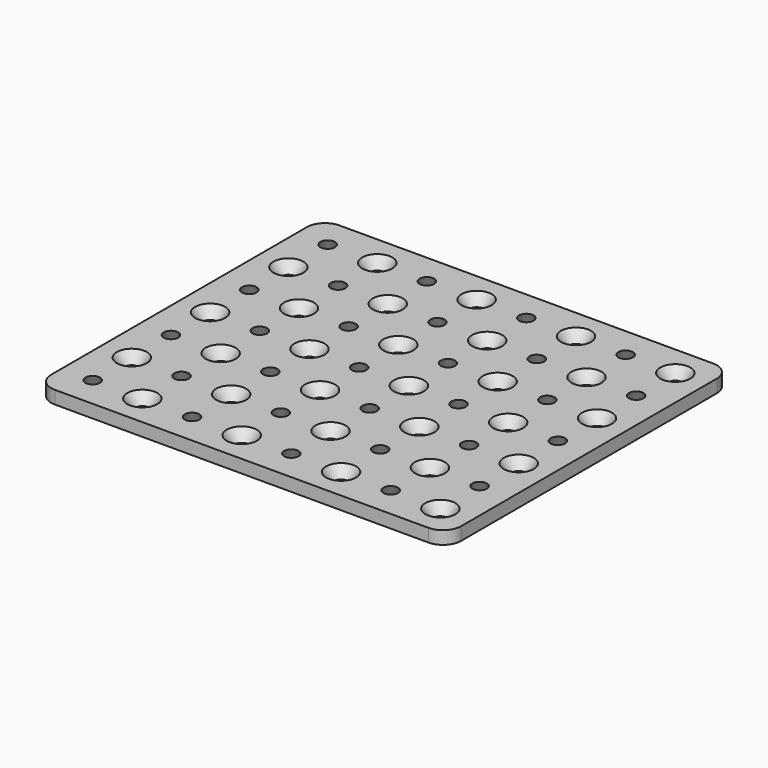
from build123d import *

# Parameters (mm, degrees)
F0_W        = 79
F0_H        = 68.58
F0_R        = 1.397
F1_DEPTH    = 1.25
F2_R        = 3.5
F3_SIZE2    = 2.49999
F3_SIZE     = 1.49999
F4_SIZE2    = 1.5
F4_SIZE     = 2
F4_2_SIZE2  = 1.5
F4_2_SIZE   = 2
F4_3_SIZE2  = 1.5
F4_3_SIZE   = 2
F4_4_SIZE2  = 1.5
F4_4_SIZE   = 2
F4_5_SIZE2  = 1.5
F4_5_SIZE   = 2
F4_6_SIZE2  = 1.5
F4_6_SIZE   = 2
F4_7_SIZE2  = 1.5
F4_7_SIZE   = 2
F4_8_SIZE2  = 1.5
F4_8_SIZE   = 2
F4_9_SIZE2  = 1.5
F4_9_SIZE   = 2
F4_10_SIZE2 = 1.5
F4_10_SIZE  = 2
F4_11_SIZE2 = 1.5
F4_11_SIZE  = 2
F4_12_SIZE2 = 1.5
F4_12_SIZE  = 2
F4_13_SIZE2 = 1.5
F4_13_SIZE  = 2
F4_14_SIZE2 = 1.5
F4_14_SIZE  = 2
F4_15_SIZE2 = 1.5
F4_15_SIZE  = 2
F4_16_SIZE2 = 1.5
F4_16_SIZE  = 2
F4_17_SIZE2 = 1.5
F4_17_SIZE  = 2
F4_18_SIZE2 = 1.5
F4_18_SIZE  = 2
F4_19_SIZE2 = 1.5
F4_19_SIZE  = 2
F4_20_SIZE2 = 1.5
F4_20_SIZE  = 2
F4_21_SIZE2 = 1.5
F4_21_SIZE  = 2
F4_22_SIZE2 = 1.5
F4_22_SIZE  = 2
F4_23_SIZE2 = 1.5
F4_23_SIZE  = 2
F4_24_SIZE2 = 1.5
F4_24_SIZE  = 2
F4_25_SIZE2 = 1.5
F4_25_SIZE  = 2
F4_26_SIZE2 = 1.5
F4_26_SIZE  = 2
F4_27_SIZE2 = 1.5
F4_27_SIZE  = 2
F4_28_SIZE2 = 1.5
F4_28_SIZE  = 2


# Not quite as in the source:
# - a fillet or chamfer is up to 0.001 mm smaller than in the source, because OpenCascade refuses the exact size


with BuildPart() as f1:
    # F0 (on Top) → F1 (new body, symmetric)
    with BuildSketch(Plane.XY):
        Rectangle(F0_W, F0_H)
        with Locations((-33.5, -28.29)):
            Circle(F0_R, mode=Mode.SUBTRACT)
        with Locations((-23.9285714286, -28.29)):
            Circle(F0_R, mode=Mode.SUBTRACT)
        with Locations((-33.5, -18.86)):
            Circle(F0_R, mode=Mode.SUBTRACT)
        with Locations((-23.9285714286, -18.86)):
            Circle(F0_R, mode=Mode.SUBTRACT)
        with Locations((-14.3571428571, -28.29)):
            Circle(F0_R, mode=Mode.SUBTRACT)
        with Locations((-4.7857142857, -28.29)):
            Circle(F0_R, mode=Mode.SUBTRACT)
        with Locations((-14.3571428571, -18.86)):
            Circle(F0_R, mode=Mode.SUBTRACT)
        with Locations((-4.7857142857, -18.86)):
            Circle(F0_R, mode=Mode.SUBTRACT)
        with Locations((-33.5, -9.43)):
            Circle(F0_R, mode=Mode.SUBTRACT)
        with Locations((-23.9285714286, -9.43)):
            Circle(F0_R, mode=Mode.SUBTRACT)
        with Locations((-14.3571428571, -9.43)):
            Circle(F0_R, mode=Mode.SUBTRACT)
        with Locations((-4.7857142857, -9.43)):
            Circle(F0_R, mode=Mode.SUBTRACT)
        with Locations((4.7857142857, -28.29)):
            Circle(F0_R, mode=Mode.SUBTRACT)
        with Locations((14.3571428571, -28.29)):
            Circle(F0_R, mode=Mode.SUBTRACT)
        with Locations((4.7857142857, -18.86)):
            Circle(F0_R, mode=Mode.SUBTRACT)
        with Locations((14.3571428571, -18.86)):
            Circle(F0_R, mode=Mode.SUBTRACT)
        with Locations((23.9285714286, -28.29)):
            Circle(F0_R, mode=Mode.SUBTRACT)
        with Locations((33.5, -28.29)):
            Circle(F0_R, mode=Mode.SUBTRACT)
        with Locations((23.9285714286, -18.86)):
            Circle(F0_R, mode=Mode.SUBTRACT)
        with Locations((33.5, -18.86)):
            Circle(F0_R, mode=Mode.SUBTRACT)
        with Locations((4.7857142857, -9.43)):
            Circle(F0_R, mode=Mode.SUBTRACT)
        with Locations((14.3571428571, -9.43)):
            Circle(F0_R, mode=Mode.SUBTRACT)
        with Locations((23.9285714286, -9.43)):
            Circle(F0_R, mode=Mode.SUBTRACT)
        with Locations((33.5, -9.43)):
            Circle(F0_R, mode=Mode.SUBTRACT)
        with Locations((-33.5, 0)):
            Circle(F0_R, mode=Mode.SUBTRACT)
        with Locations((-23.9285714286, 0)):
            Circle(F0_R, mode=Mode.SUBTRACT)
        with Locations((-33.5, 9.43)):
            Circle(F0_R, mode=Mode.SUBTRACT)
        with Locations((-23.9285714286, 9.43)):
            Circle(F0_R, mode=Mode.SUBTRACT)
        with Locations((-14.3571428571, 0)):
            Circle(F0_R, mode=Mode.SUBTRACT)
        with Locations((-4.7857142857, 0)):
            Circle(F0_R, mode=Mode.SUBTRACT)
        with Locations((-14.3571428571, 9.43)):
            Circle(F0_R, mode=Mode.SUBTRACT)
        with Locations((-4.7857142857, 9.43)):
            Circle(F0_R, mode=Mode.SUBTRACT)
        with Locations((-33.5, 18.86)):
            Circle(F0_R, mode=Mode.SUBTRACT)
        with Locations((-23.9285714286, 18.86)):
            Circle(F0_R, mode=Mode.SUBTRACT)
        with Locations((-33.5, 28.29)):
            Circle(F0_R, mode=Mode.SUBTRACT)
        with Locations((-23.9285714286, 28.29)):
            Circle(F0_R, mode=Mode.SUBTRACT)
        with Locations((-14.3571428571, 18.86)):
            Circle(F0_R, mode=Mode.SUBTRACT)
        with Locations((-4.7857142857, 18.86)):
            Circle(F0_R, mode=Mode.SUBTRACT)
        with Locations((-14.3571428571, 28.29)):
            Circle(F0_R, mode=Mode.SUBTRACT)
        with Locations((-4.7857142857, 28.29)):
            Circle(F0_R, mode=Mode.SUBTRACT)
        with Locations((4.7857142857, 0)):
            Circle(F0_R, mode=Mode.SUBTRACT)
        with Locations((14.3571428571, 0)):
            Circle(F0_R, mode=Mode.SUBTRACT)
        with Locations((4.7857142857, 9.43)):
            Circle(F0_R, mode=Mode.SUBTRACT)
        with Locations((14.3571428571, 9.43)):
            Circle(F0_R, mode=Mode.SUBTRACT)
        with Locations((23.9285714286, 0)):
            Circle(F0_R, mode=Mode.SUBTRACT)
        with Locations((33.5, 0)):
            Circle(F0_R, mode=Mode.SUBTRACT)
        with Locations((23.9285714286, 9.43)):
            Circle(F0_R, mode=Mode.SUBTRACT)
        with Locations((33.5, 9.43)):
            Circle(F0_R, mode=Mode.SUBTRACT)
        with Locations((4.7857142857, 18.86)):
            Circle(F0_R, mode=Mode.SUBTRACT)
        with Locations((14.3571428571, 18.86)):
            Circle(F0_R, mode=Mode.SUBTRACT)
        with Locations((4.7857142857, 28.29)):
            Circle(F0_R, mode=Mode.SUBTRACT)
        with Locations((14.3571428571, 28.29)):
            Circle(F0_R, mode=Mode.SUBTRACT)
        with Locations((23.9285714286, 18.86)):
            Circle(F0_R, mode=Mode.SUBTRACT)
        with Locations((33.5, 18.86)):
            Circle(F0_R, mode=Mode.SUBTRACT)
        with Locations((23.9285714286, 28.29)):
            Circle(F0_R, mode=Mode.SUBTRACT)
        with Locations((33.5, 28.29)):
            Circle(F0_R, mode=Mode.SUBTRACT)
    extrude(amount=F1_DEPTH, both=True)

    # F2
    f2_edges = [f1.edges().sort_by_distance(p)[0] for p in [
        (39.5, -34.29, 0),
        (-39.5, -34.29, 0),
        (-39.5, 34.29, 0),
        (39.5, 34.29, 0),
    ]]
    fillet(f2_edges, radius=F2_R)

    # F3 (size 1.5 and 2.5 in the source; OpenCascade refuses exactly that, so slightly less here)
    f3_edges = [f1.edges().sort_by_distance(p)[0] for p in [
        (-15.754143, 28.29, -1.25),
        (-25.325571, 18.86, -1.25),
        (-34.897, 9.43, -1.25),
        (3.388714, 28.29, -1.25),
        (-6.182714, 18.86, -1.25),
        (-15.754143, 9.43, -1.25),
        (-25.325571, 0, -1.25),
        (-34.897, -9.43, -1.25),
        (-34.897, -28.29, -1.25),
        (-25.325571, -18.86, -1.25),
        (-15.754143, -9.43, -1.25),
        (-6.182714, 0, -1.25),
        (3.388714, 9.43, -1.25),
        (12.960143, 18.86, -1.25),
        (22.531571, 28.29, -1.25),
        (32.103, 18.86, -1.25),
        (12.960143, 0, -1.25),
        (3.388714, -9.43, -1.25),
        (-6.182714, -18.86, -1.25),
        (-15.754143, -28.29, -1.25),
        (32.103, 0, -1.25),
        (22.531571, -9.43, -1.25),
        (12.960143, -18.86, -1.25),
        (3.388714, -28.29, -1.25),
        (32.103, -18.86, -1.25),
        (22.531571, -28.29, -1.25),
        (22.531571, 9.43, -1.25),
        (-34.897, 28.29, -1.25),
    ]]
    f3_side = f1.faces().sort_by_distance((0, 0, -1.25))[0]
    chamfer(f3_edges, length=F3_SIZE, length2=F3_SIZE2, reference=f3_side)

    # F4
    f4_edges = [f1.edges().sort_by_distance(p)[0] for p in [
        (-25.325571, 28.29, 1.25),
    ]]
    f4_side = f1.faces().sort_by_distance((-25.325571, 28.29, 0))[0]
    chamfer(f4_edges, length=F4_SIZE, length2=F4_SIZE2, reference=f4_side)

    # F4#2
    f4_2_edges = [f1.edges().sort_by_distance(p)[0] for p in [
        (-34.897, 0, 1.25),
    ]]
    f4_2_side = f1.faces().sort_by_distance((-34.897, 0, 0))[0]
    chamfer(f4_2_edges, length=F4_2_SIZE, length2=F4_2_SIZE2, reference=f4_2_side)

    # F4#3
    f4_3_edges = [f1.edges().sort_by_distance(p)[0] for p in [
        (-25.325571, 9.43, 1.25),
    ]]
    f4_3_side = f1.faces().sort_by_distance((-25.325571, 9.43, 0))[0]
    chamfer(f4_3_edges, length=F4_3_SIZE, length2=F4_3_SIZE2, reference=f4_3_side)

    # F4#4
    f4_4_edges = [f1.edges().sort_by_distance(p)[0] for p in [
        (-15.754143, 18.86, 1.25),
    ]]
    f4_4_side = f1.faces().sort_by_distance((-15.754143, 18.86, 0))[0]
    chamfer(f4_4_edges, length=F4_4_SIZE, length2=F4_4_SIZE2, reference=f4_4_side)

    # F4#5
    f4_5_edges = [f1.edges().sort_by_distance(p)[0] for p in [
        (-6.182714, 28.29, 1.25),
    ]]
    f4_5_side = f1.faces().sort_by_distance((-6.182714, 28.29, 0))[0]
    chamfer(f4_5_edges, length=F4_5_SIZE, length2=F4_5_SIZE2, reference=f4_5_side)

    # F4#6
    f4_6_edges = [f1.edges().sort_by_distance(p)[0] for p in [
        (-34.897, -18.86, 1.25),
    ]]
    f4_6_side = f1.faces().sort_by_distance((-34.897, -18.86, 0))[0]
    chamfer(f4_6_edges, length=F4_6_SIZE, length2=F4_6_SIZE2, reference=f4_6_side)

    # F4#7
    f4_7_edges = [f1.edges().sort_by_distance(p)[0] for p in [
        (-25.325571, -9.43, 1.25),
    ]]
    f4_7_side = f1.faces().sort_by_distance((-25.325571, -9.43, 0))[0]
    chamfer(f4_7_edges, length=F4_7_SIZE, length2=F4_7_SIZE2, reference=f4_7_side)

    # F4#8
    f4_8_edges = [f1.edges().sort_by_distance(p)[0] for p in [
        (-15.754143, 0, 1.25),
    ]]
    f4_8_side = f1.faces().sort_by_distance((-15.754143, 0, 0))[0]
    chamfer(f4_8_edges, length=F4_8_SIZE, length2=F4_8_SIZE2, reference=f4_8_side)

    # F4#9
    f4_9_edges = [f1.edges().sort_by_distance(p)[0] for p in [
        (-6.182714, 9.43, 1.25),
    ]]
    f4_9_side = f1.faces().sort_by_distance((-6.182714, 9.43, 0))[0]
    chamfer(f4_9_edges, length=F4_9_SIZE, length2=F4_9_SIZE2, reference=f4_9_side)

    # F4#10
    f4_10_edges = [f1.edges().sort_by_distance(p)[0] for p in [
        (3.388714, 18.86, 1.25),
    ]]
    f4_10_side = f1.faces().sort_by_distance((3.388714, 18.86, 0))[0]
    chamfer(f4_10_edges, length=F4_10_SIZE, length2=F4_10_SIZE2, reference=f4_10_side)

    # F4#11
    f4_11_edges = [f1.edges().sort_by_distance(p)[0] for p in [
        (12.960143, 28.29, 1.25),
    ]]
    f4_11_side = f1.faces().sort_by_distance((12.960143, 28.29, 0))[0]
    chamfer(f4_11_edges, length=F4_11_SIZE, length2=F4_11_SIZE2, reference=f4_11_side)

    # F4#12
    f4_12_edges = [f1.edges().sort_by_distance(p)[0] for p in [
        (22.531571, 18.86, 1.25),
    ]]
    f4_12_side = f1.faces().sort_by_distance((22.531571, 18.86, 0))[0]
    chamfer(f4_12_edges, length=F4_12_SIZE, length2=F4_12_SIZE2, reference=f4_12_side)

    # F4#13
    f4_13_edges = [f1.edges().sort_by_distance(p)[0] for p in [
        (32.103, 28.29, 1.25),
    ]]
    f4_13_side = f1.faces().sort_by_distance((32.103, 28.29, 0))[0]
    chamfer(f4_13_edges, length=F4_13_SIZE, length2=F4_13_SIZE2, reference=f4_13_side)

    # F4#14
    f4_14_edges = [f1.edges().sort_by_distance(p)[0] for p in [
        (12.960143, 9.43, 1.25),
    ]]
    f4_14_side = f1.faces().sort_by_distance((12.960143, 9.43, 0))[0]
    chamfer(f4_14_edges, length=F4_14_SIZE, length2=F4_14_SIZE2, reference=f4_14_side)

    # F4#15
    f4_15_edges = [f1.edges().sort_by_distance(p)[0] for p in [
        (3.388714, 0, 1.25),
    ]]
    f4_15_side = f1.faces().sort_by_distance((3.388714, 0, 0))[0]
    chamfer(f4_15_edges, length=F4_15_SIZE, length2=F4_15_SIZE2, reference=f4_15_side)

    # F4#16
    f4_16_edges = [f1.edges().sort_by_distance(p)[0] for p in [
        (-6.182714, -9.43, 1.25),
    ]]
    f4_16_side = f1.faces().sort_by_distance((-6.182714, -9.43, 0))[0]
    chamfer(f4_16_edges, length=F4_16_SIZE, length2=F4_16_SIZE2, reference=f4_16_side)

    # F4#17
    f4_17_edges = [f1.edges().sort_by_distance(p)[0] for p in [
        (-15.754143, -18.86, 1.25),
    ]]
    f4_17_side = f1.faces().sort_by_distance((-15.754143, -18.86, 0))[0]
    chamfer(f4_17_edges, length=F4_17_SIZE, length2=F4_17_SIZE2, reference=f4_17_side)

    # F4#18
    f4_18_edges = [f1.edges().sort_by_distance(p)[0] for p in [
        (-25.325571, -28.29, 1.25),
    ]]
    f4_18_side = f1.faces().sort_by_distance((-25.325571, -28.29, 0))[0]
    chamfer(f4_18_edges, length=F4_18_SIZE, length2=F4_18_SIZE2, reference=f4_18_side)

    # F4#19
    f4_19_edges = [f1.edges().sort_by_distance(p)[0] for p in [
        (22.531571, 0, 1.25),
    ]]
    f4_19_side = f1.faces().sort_by_distance((22.531571, 0, 0))[0]
    chamfer(f4_19_edges, length=F4_19_SIZE, length2=F4_19_SIZE2, reference=f4_19_side)

    # F4#20
    f4_20_edges = [f1.edges().sort_by_distance(p)[0] for p in [
        (32.103, -9.43, 1.25),
    ]]
    f4_20_side = f1.faces().sort_by_distance((32.103, -9.43, 0))[0]
    chamfer(f4_20_edges, length=F4_20_SIZE, length2=F4_20_SIZE2, reference=f4_20_side)

    # F4#21
    f4_21_edges = [f1.edges().sort_by_distance(p)[0] for p in [
        (32.103, 9.43, 1.25),
    ]]
    f4_21_side = f1.faces().sort_by_distance((32.103, 9.43, 0))[0]
    chamfer(f4_21_edges, length=F4_21_SIZE, length2=F4_21_SIZE2, reference=f4_21_side)

    # F4#22
    f4_22_edges = [f1.edges().sort_by_distance(p)[0] for p in [
        (12.960143, -9.43, 1.25),
    ]]
    f4_22_side = f1.faces().sort_by_distance((12.960143, -9.43, 0))[0]
    chamfer(f4_22_edges, length=F4_22_SIZE, length2=F4_22_SIZE2, reference=f4_22_side)

    # F4#23
    f4_23_edges = [f1.edges().sort_by_distance(p)[0] for p in [
        (22.531571, -18.86, 1.25),
    ]]
    f4_23_side = f1.faces().sort_by_distance((22.531571, -18.86, 0))[0]
    chamfer(f4_23_edges, length=F4_23_SIZE, length2=F4_23_SIZE2, reference=f4_23_side)

    # F4#24
    f4_24_edges = [f1.edges().sort_by_distance(p)[0] for p in [
        (32.103, -28.29, 1.25),
    ]]
    f4_24_side = f1.faces().sort_by_distance((32.103, -28.29, 0))[0]
    chamfer(f4_24_edges, length=F4_24_SIZE, length2=F4_24_SIZE2, reference=f4_24_side)

    # F4#25
    f4_25_edges = [f1.edges().sort_by_distance(p)[0] for p in [
        (3.388714, -18.86, 1.25),
    ]]
    f4_25_side = f1.faces().sort_by_distance((3.388714, -18.86, 0))[0]
    chamfer(f4_25_edges, length=F4_25_SIZE, length2=F4_25_SIZE2, reference=f4_25_side)

    # F4#26
    f4_26_edges = [f1.edges().sort_by_distance(p)[0] for p in [
        (12.960143, -28.29, 1.25),
    ]]
    f4_26_side = f1.faces().sort_by_distance((12.960143, -28.29, 0))[0]
    chamfer(f4_26_edges, length=F4_26_SIZE, length2=F4_26_SIZE2, reference=f4_26_side)

    # F4#27
    f4_27_edges = [f1.edges().sort_by_distance(p)[0] for p in [
        (-6.182714, -28.29, 1.25),
    ]]
    f4_27_side = f1.faces().sort_by_distance((-6.182714, -28.29, 0))[0]
    chamfer(f4_27_edges, length=F4_27_SIZE, length2=F4_27_SIZE2, reference=f4_27_side)

    # F4#28
    f4_28_edges = [f1.edges().sort_by_distance(p)[0] for p in [
        (-34.897, 18.86, 1.25),
    ]]
    f4_28_side = f1.faces().sort_by_distance((-34.897, 18.86, 0))[0]
    chamfer(f4_28_edges, length=F4_28_SIZE, length2=F4_28_SIZE2, reference=f4_28_side)


solid = f1.part
